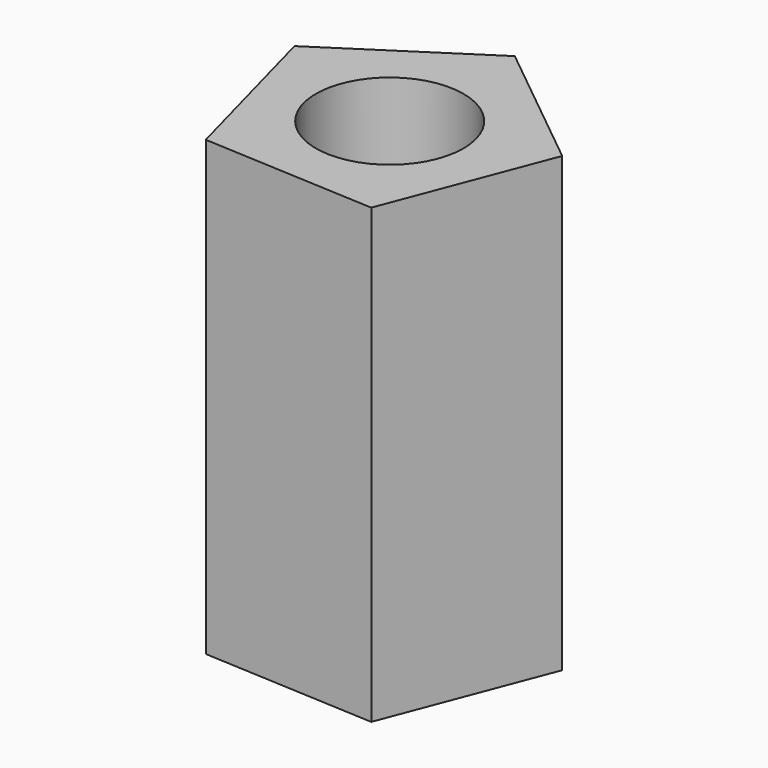
from build123d import *

# Parameters (mm, degrees)
F4_R     = 13.2572976872
F5_DEPTH = 40.64


# Not quite as in the source:
# - the program builds the solid bodies; features that only make, move or delete a surface that nothing else refers to are left out


with BuildPart() as f5:
    # F4 (on Top) → F5 (new body, symmetric)
    with BuildSketch(Plane.XY):
        Polygon((-11.3957837711, 9.4445306856), (-3.343205899, -20.527953282), (27.650703699, -22.1315035333), (38.7534154026, 6.8499318763), (14.6213590048, 26.3649942535), align=None)
        with Locations((13.2572976872, 0)):
            Circle(F4_R, mode=Mode.SUBTRACT)
    extrude(amount=F5_DEPTH, both=True)


solid = f5.part
